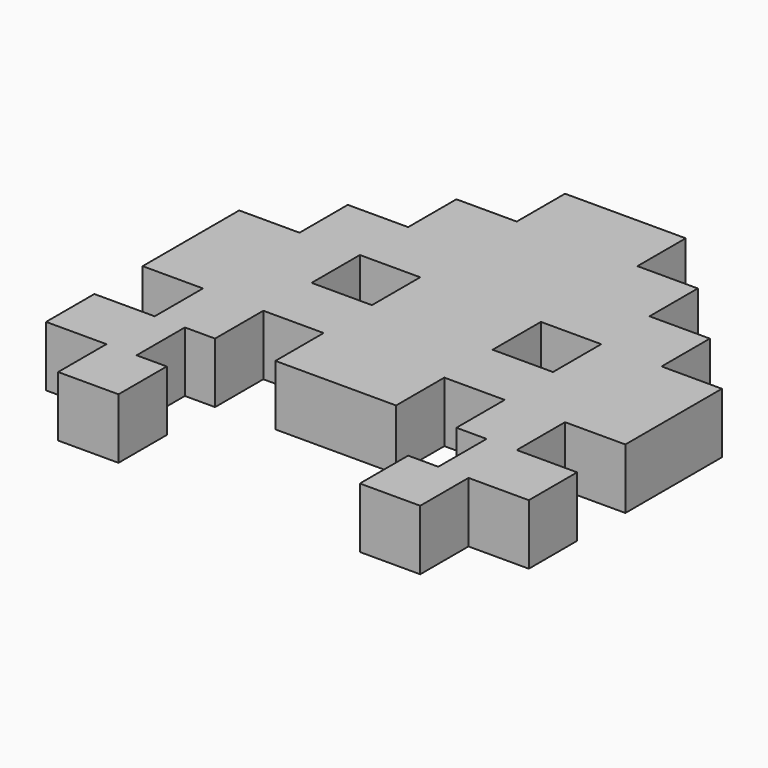
from build123d import *

# Parameters (mm, degrees)
F0_W     = 10
F0_H     = 10
F0_R     = 6
F1_DEPTH = 10
F3_DEPTH = 3


with BuildPart() as f1:
    # F0 (on Top) → F1 (new body)
    with BuildSketch(Plane.XY):
        Polygon((10, 0), (0, 0), (-10, 0), (-10, -10), (-20, -10), (-20, -20), (-30, -20), (-30, -30), (-40, -30), (-40, -40), (-40, -50), (-30, -50), (-30, -60), (-40, -60), (-40, -70), (-30, -70), (-30, -80), (-20, -80), (-20, -70), (-25, -70), (-25, -60), (-20, -60), (-20, -50), (-10, -50), (-10, -60), (0, -60), (10, -60), (10, -50), (20, -50), (20, -60), (25, -60), (25, -70), (20, -70), (20, -80), (30, -80), (30, -70), (40, -70), (40, -60), (30, -60), (30, -50), (40, -50), (40, -40), (40, -30), (30, -30), (30, -20), (20, -20), (20, -10), (10, -10), align=None)
        with Locations((-15, -35)):
            Rectangle(F0_W, F0_H, mode=Mode.SUBTRACT)
        with Locations((15, -35)):
            Rectangle(F0_W, F0_H, mode=Mode.SUBTRACT)
        with Locations((0, -15)):
            Circle(F0_R, mode=Mode.SUBTRACT)
        with Locations((0, -15)):
            Circle(F0_R)
    extrude(amount=F1_DEPTH)

    # F2 (on Right) → F3 (cut, symmetric)
    with BuildSketch(Plane.YZ):
        Polygon((-30, 5), (-30, 0), (-24, 0), (-21.1132486541, 5), align=None)
    extrude(amount=F3_DEPTH, both=True, mode=Mode.SUBTRACT)


solid = f1.part
